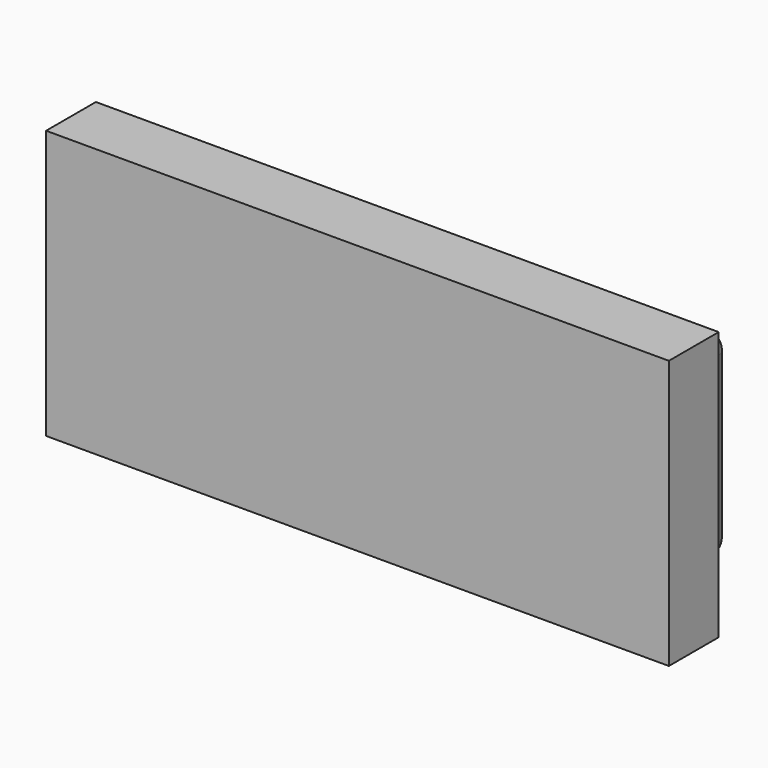
from build123d import *

# Parameters (mm, degrees)
F0_W     = 199.9996
F0_H     = 86.2838
F1_DEPTH = 19.9898
F2_W     = 175.8382518563
F2_H     = 63.7771419656
F3_DEPTH = 19.9898
F4_R     = 5.5188922036


# Not quite as in the source:
# - the program builds the solid bodies; features that only make, move or delete a surface that nothing else refers to are left out


with BuildPart() as f1:
    # F0 (on Front) → F1 (new body)
    with BuildSketch(Plane.XZ):
        with Locations((27.3758191615, -15.038352045)):
            Rectangle(F0_W, F0_H)
    extrude(amount=F1_DEPTH)

    # F2 (on face) → F3 (join)
    with BuildSketch(Plane(origin=(0, 0, 0), x_dir=(-1, 0, 0), z_dir=(0, 1, 0))):
        with Locations((-27.3758191615, -15.038352045)):
            Rectangle(F2_W, F2_H)
    extrude(amount=F3_DEPTH)

    # F4
    f4_edges = [f1.edges().sort_by_distance(p)[0] for p in [
        (-60.543307, 9.9949, 16.850219),
        (115.294945, 9.9949, 16.850219),
        (27.375819, 0, 16.850219),
        (27.375819, 19.9898, 16.850219),
        (115.294945, 9.9949, -46.926923),
        (-60.543307, 9.9949, -46.926923),
        (27.375819, 0, -46.926923),
        (27.375819, 19.9898, -46.926923),
        (-60.543307, 0, -15.038352),
        (-60.543307, 19.9898, -15.038352),
        (115.294945, 0, -15.038352),
        (115.294945, 19.9898, -15.038352),
    ]]
    fillet(f4_edges, radius=F4_R)


solid = f1.part
